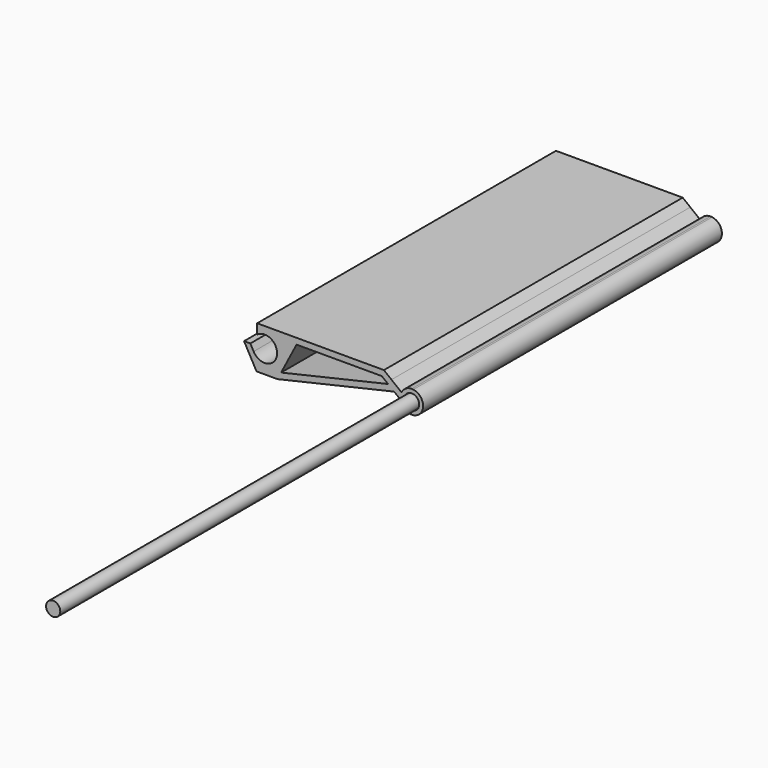
from build123d import *

# Parameters (mm, degrees)
F0_R     = 2
F1_DEPTH = 100
F0_R_2   = 1.9
F2_DEPTH = 220


# Not quite as in the source:
# - a feature names something its author has since deleted; it is built from what else it names


with BuildPart() as f1:
    # F0 (on Front) → F1 (new body)
    with BuildSketch(Plane.XZ):
        with BuildLine():
            Line((31.3843597952, 3.75), (33.9666413399, 3.75))
            Line((33.9666413399, 3.75), (31.9397772655, 5.35))
            Line((31.9397772655, 5.35), (9.3864129766, 5.35))
            Line((9.3864129766, 5.35), (0, 5.35))
            Line((0, 5.35), (0, 3.35))
            ThreePointArc((0, 3.35), (2.8827538929, -1.7065257082), (-2.9370111217, -1.6113552281))
            Line((-2.9370111217, -1.6113552281), (-3.8210614584, 0))
            Line((-3.8210614584, 0), (-5.5, 0))
            Line((-5.5, 0), (-2.1625379435, -6.05))
            Line((-2.1625379435, -6.05), (3.4431787948, -6.05))
            Line((3.4431787948, -6.05), (4.4164381013, -4.1831450595))
            Line((4.4164381013, -4.1831450595), (8.5522748458, 3.75))
            Line((8.5522748458, 3.75), (31.3843597952, 3.75))
        make_face()
        with BuildLine():
            ThreePointArc((36.3761074084, -0.1904695569), (36.368841785, 0.7435810003), (36.6446012215, 1.6360270579))
            Line((36.6446012215, 1.6360270579), (33.9666413399, 3.75))
            Line((33.9666413399, 3.75), (31.3843597952, 3.75))
            Line((31.3843597952, 3.75), (33.0560092942, 2.4304052467))
            Line((33.0560092942, 2.4304052467), (34.6654122242, 1.1599477351))
            Line((34.6654122242, 1.1599477351), (36.3761074084, -0.1904695569))
        make_face()
        with BuildLine():
            ThreePointArc((38.1222629657, 3.0756845552), (37.4249855205, 2.6356588652), (36.8710474529, 2.0249452984))
            ThreePointArc((36.8710474529, 2.0249452984), (36.7506412519, 1.8346685035), (36.6446012215, 1.6360270579))
            ThreePointArc((36.6446012215, 1.6360270579), (36.368841785, 0.7435810003), (36.3761074084, -0.1904695569))
            ThreePointArc((36.3761074084, -0.1904695569), (41.5647564685, -1.8347879593), (39.8159904414, 3.3195965296))
            ThreePointArc((39.8159904414, 3.3195965296), (39.6017389906, 3.3423896377), (39.3864129766, 3.35))
            ThreePointArc((39.3864129766, 3.35), (38.7396278087, 3.2806323065), (38.1222629657, 3.0756845552))
        make_face()
        with Locations((39.3864129766, 0.3)):
            Circle(F0_R, mode=Mode.SUBTRACT)
        Polygon((3.4431787948, -6.05), (34.6654122242, 1.1599477351), (33.0560092942, 2.4304052467), (4.4164381013, -4.1831450595), align=None)
        with BuildLine():
            Line((0, 3.35), (0, 5.35))
            Line((0, 5.35), (-2, 5.35))
            Line((-2, 5.35), (-2, 2.6874709301))
            ThreePointArc((-2, 2.6874709301), (-1.0534401702, 3.180057202), (0, 3.35))
        make_face()
    extrude(amount=F1_DEPTH)


with BuildPart() as f2:
    # F0 (on Front) → F2 (new body)
    with BuildSketch(Plane.XZ):
        with Locations((39.3864129766, 0.3)):
            Circle(F0_R_2)
    extrude(amount=F2_DEPTH)


solid = Compound([f1.part, f2.part])
